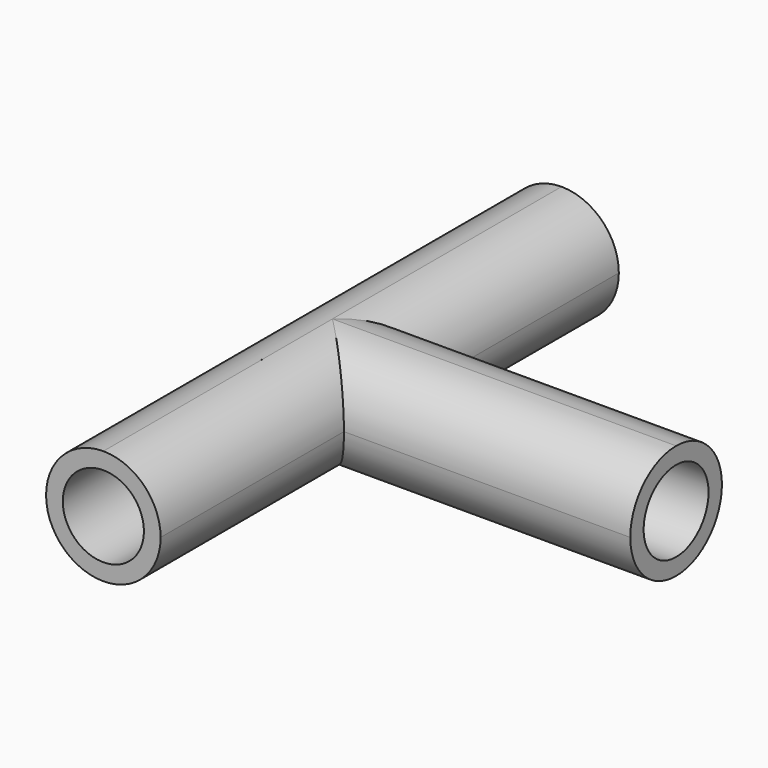
from build123d import *

# Parameters (mm, degrees)
F0_W     = 30
F0_H     = 6
F1_DEPTH = 12
F3_R     = 4.25
F5_DEPTH = 20
F4_R     = 4.25
F6_DEPTH = 20
F2_R     = 4.25
F7_DEPTH = 20
F8_R     = 5.99999


# Not quite as in the source:
# - a fillet or chamfer is up to 0.001 mm smaller than in the source, because OpenCascade refuses the exact size


with BuildPart() as f1:
    # F0 (on Top) → F1 (new body)
    with BuildSketch(Plane.XY):
        Polygon((-6, -30), (6, -30), (6, -6), (6, 0), (6, 6), (6, 30), (0, 30), (-6, 30), align=None)
        with Locations((21, 3)):
            Rectangle(F0_W, F0_H)
        with Locations((21, -3)):
            Rectangle(F0_W, F0_H)
    extrude(amount=F1_DEPTH)

    # F3 (on face) → F5 (cut)
    with BuildSketch(Plane(origin=(0, 30, 0), x_dir=(-1, 0, 0), z_dir=(0, 1, 0))):
        with Locations((0, 6)):
            Circle(F3_R)
    extrude(amount=-F5_DEPTH, mode=Mode.SUBTRACT)

    # F4 (on face) → F6 (cut)
    with BuildSketch(Plane.XZ.offset(30)):
        with Locations((0, 6)):
            Circle(F4_R)
    extrude(amount=-F6_DEPTH, mode=Mode.SUBTRACT)

    # F2 (on face) → F7 (cut)
    with BuildSketch(Plane.YZ.offset(36)):
        with Locations((0, 6)):
            Circle(F2_R)
    extrude(amount=-F7_DEPTH, mode=Mode.SUBTRACT)

    # F8 (radius 6 in the source; OpenCascade refuses exactly that, so slightly less here)
    f8_edges = [f1.edges().sort_by_distance(p)[0] for p in [
        (6, -18, 12),
        (21, -6, 12),
        (21, 6, 12),
        (6, 18, 12),
        (-6, 0, 12),
        (-6, 0, 0),
        (6, 18, 0),
        (6, -18, 0),
        (21, -6, 0),
        (21, 6, 0),
    ]]
    fillet(f8_edges, radius=F8_R)


solid = f1.part
